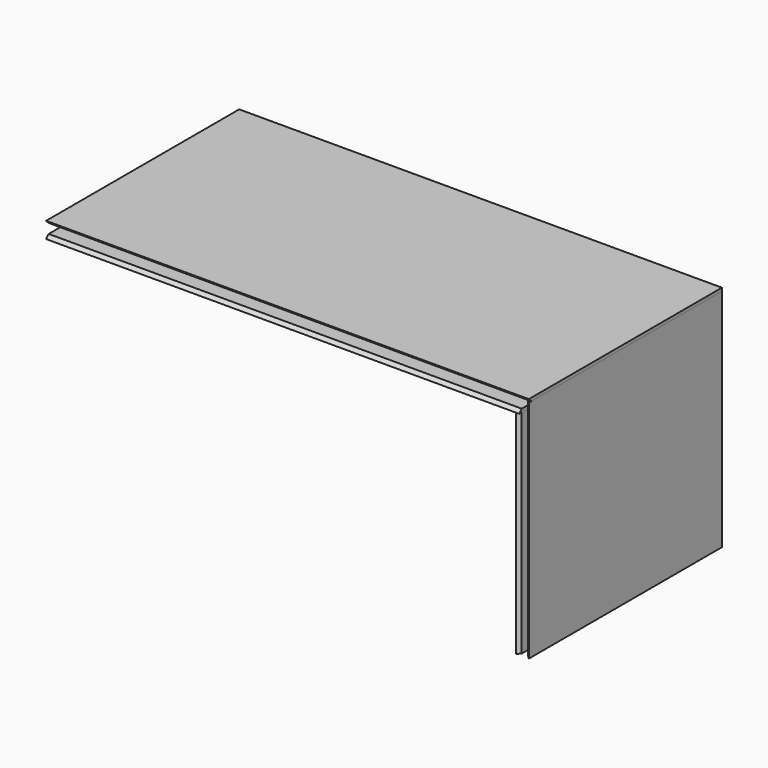
from build123d import *

# Parameters (mm, degrees)
F3_W      = 1500
F3_H      = 10
F7_DEPTH  = 750
F4_W      = 1470
F4_H      = 10
F8_DEPTH  = 750
F5_W      = 10
F5_H      = 700
F9_DEPTH  = 750
F6_W      = 10
F6_H      = 660
F10_DEPTH = 750
F11_SIZE  = 9.99999
F12_SIZE  = 9.99999
F13_SIZE  = 9.99999
F14_SIZE  = 9.99999


# Not quite as in the source:
# - a fillet or chamfer is up to 0.001 mm smaller than in the source, because OpenCascade refuses the exact size


with BuildPart() as f7:
    # F3 (on face) → F7 (new body)
    with BuildSketch(Plane.XZ):
        with Locations((-515, 705)):
            Rectangle(F3_W, F3_H)
    extrude(amount=F7_DEPTH)

    # F11 (size 10 in the source; OpenCascade refuses exactly that, so slightly less here)
    f11_edges = [f7.edges().sort_by_distance(p)[0] for p in [
        (-515, -750, 700),
    ]]
    chamfer(f11_edges, length=F11_SIZE)


with BuildPart() as f8:
    # F4 (on face) → F8 (new body)
    with BuildSketch(Plane.XZ):
        with Locations((-530, 665)):
            Rectangle(F4_W, F4_H)
    extrude(amount=F8_DEPTH)

    # F12 (size 10 in the source; OpenCascade refuses exactly that, so slightly less here)
    f12_edges = [f8.edges().sort_by_distance(p)[0] for p in [
        (-530, -750, 670),
    ]]
    chamfer(f12_edges, length=F12_SIZE)


with BuildPart() as f9:
    # F5 (on face) → F9 (new body)
    with BuildSketch(Plane.XZ):
        with Locations((230, 350)):
            Rectangle(F5_W, F5_H)
    extrude(amount=F9_DEPTH)

    # F14 (size 10 in the source; OpenCascade refuses exactly that, so slightly less here)
    f14_edges = [f9.edges().sort_by_distance(p)[0] for p in [
        (225, -750, 350),
    ]]
    chamfer(f14_edges, length=F14_SIZE)


with BuildPart() as f10:
    # F6 (on face) → F10 (new body)
    with BuildSketch(Plane.XZ):
        with Locations((200, 330)):
            Rectangle(F6_W, F6_H)
    extrude(amount=F10_DEPTH)

    # F13 (size 10 in the source; OpenCascade refuses exactly that, so slightly less here)
    f13_edges = [f10.edges().sort_by_distance(p)[0] for p in [
        (205, -750, 330),
    ]]
    chamfer(f13_edges, length=F13_SIZE)


solid = Compound([f7.part, f8.part, f9.part, f10.part])
